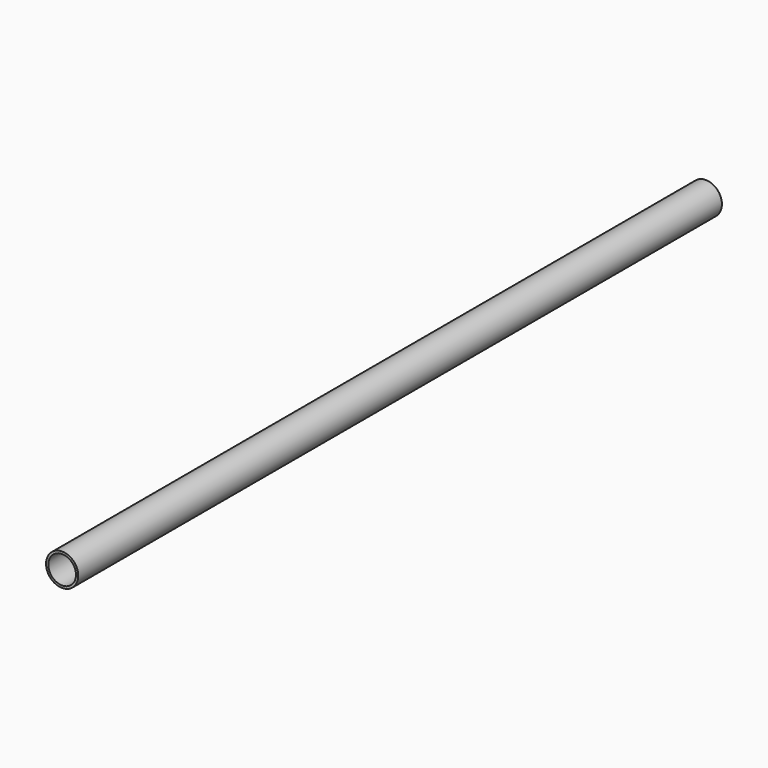
from build123d import *

# Parameters (mm, degrees)
F0_R     = 6.35
F1_DEPTH = 158.75
F2_T     = -0.889


with BuildPart() as f1:
    # F0 (on Front) → F1 (new body, symmetric)
    with BuildSketch(Plane.XZ):
        with Locations((0, 1.314903493)):
            Circle(F0_R)
    extrude(amount=F1_DEPTH, both=True)

    # F2
    f2_openings = [f1.faces().sort_by_distance(p)[0] for p in [
        (0, -158.75, 1.314903),
        (0, 158.75, 1.314903),
    ]]
    offset(amount=F2_T, openings=f2_openings)


solid = f1.part
